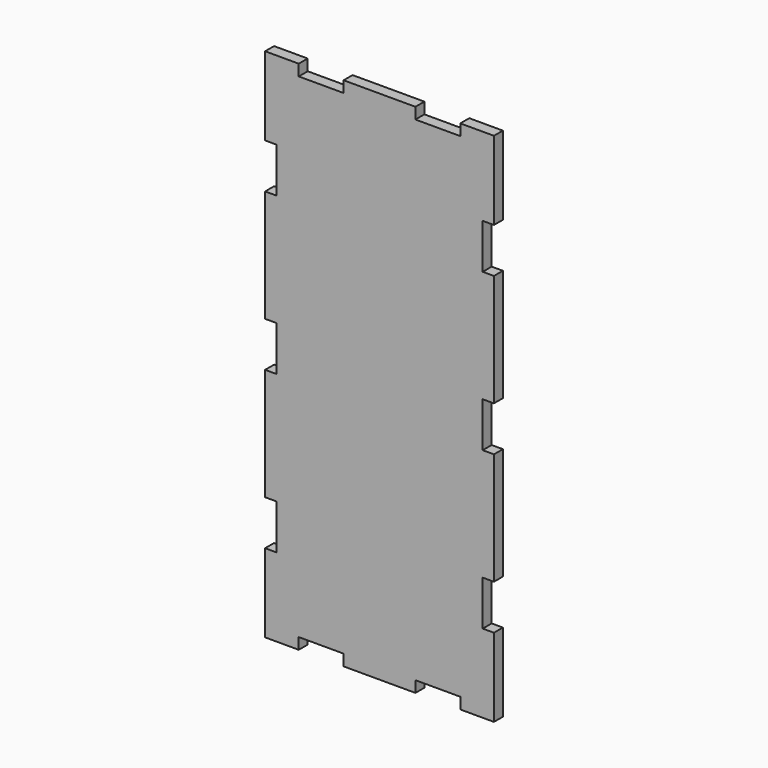
from build123d import *

# Parameters (mm, degrees)
F1_DEPTH = 3.175


# Not quite as in the source:
# - a feature names something its author has since deleted; it is built from what else it names


with BuildPart() as f1:
    # F0 (on Front) → F1 (new body)
    with BuildSketch(Plane.XZ):
        Polygon((-31.2676696369, 73.66), (-31.2676696369, 51.435), (-28.0926696369, 51.435), (-28.0926696369, 38.735), (-31.2676696369, 38.735), (-31.2676696369, 6.985), (-28.0926696369, 6.985), (-28.0926696369, -5.715), (-31.2676696369, -5.715), (-31.2676696369, -37.465), (-28.0926696369, -37.465), (-28.0926696369, -50.165), (-31.2676696369, -50.165), (-31.2676696369, -72.39), (-21.7426696369, -72.39), (-21.7426696369, -69.215), (-9.0426696369, -69.215), (-9.0426696369, -72.39), (11.2773303631, -72.39), (11.2773303631, -69.215), (23.9773303631, -69.215), (23.9773303631, -72.39), (33.5023303631, -72.39), (33.5023303631, -50.165), (30.3273303631, -50.165), (30.3273303631, -37.465), (33.5023303631, -37.465), (33.5023303631, -5.715), (30.3273303631, -5.715), (30.3273303631, 6.985), (33.5023303631, 6.985), (33.5023303631, 38.735), (30.3273303631, 38.735), (30.3273303631, 51.435), (33.5023303631, 51.435), (33.5023303631, 73.66), (23.9773303631, 73.66), (23.9773303631, 70.485), (11.2773303631, 70.485), (11.2773303631, 73.66), (-9.0426696369, 73.66), (-9.0426696369, 70.485), (-21.7426696369, 70.485), (-21.7426696369, 73.66), align=None)
    extrude(amount=F1_DEPTH)


solid = f1.part
